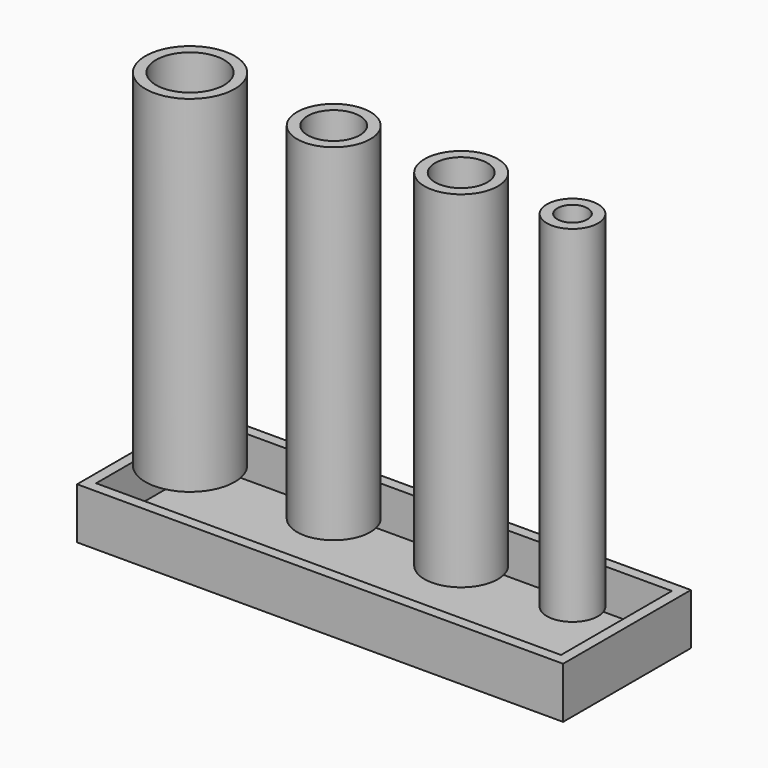
from build123d import *

# Parameters (mm, degrees)
F0_R     = 10.721612753
F1_DEPTH = 83.058
F0_R_2   = 8.8103259694
F0_R_3   = 8.8179558516
F0_R_4   = 6.164722253
F2_W     = 116.6835911572
F2_H     = 12.2901778668
F3_DEPTH = 19.177
F4_T     = -2.54
F4_2_T   = -2.54
F4_3_T   = -2.54
F4_4_T   = -2.54
F5_T     = -2.54


# Not quite as in the source:
# - a feature names something its author has since deleted; it is built from what else it names


with BuildPart() as f1:
    # F0 (on Top) → F1 (new body)
    with BuildSketch(Plane.XY):
        with Locations((-50.1845553517, 0)):
            Circle(F0_R)
    extrude(amount=F1_DEPTH)

    # F4
    f4_openings = [f1.faces().sort_by_distance(p)[0] for p in [
        (-50.184555, 0, 83.058),
    ]]
    offset(amount=F4_T, openings=f4_openings)


with BuildPart() as f1b:
    # F0 (on Top) → F1, piece 2 (new body)
    with BuildSketch(Plane.XY):
        with Locations((-15.6907774508, 0)):
            Circle(F0_R_2)
    extrude(amount=F1_DEPTH)

    # F4#4
    f4_4_openings = [f1b.faces().sort_by_distance(p)[0] for p in [
        (-15.690777, 0, 83.058),
    ]]
    offset(amount=F4_4_T, openings=f4_4_openings)


with BuildPart() as f1c:
    # F0 (on Top) → F1, piece 3 (new body)
    with BuildSketch(Plane.XY):
        with Locations((14.9127244949, 0)):
            Circle(F0_R_3)
    extrude(amount=F1_DEPTH)

    # F4#2
    f4_2_openings = [f1c.faces().sort_by_distance(p)[0] for p in [
        (14.912724, 0, 83.058),
    ]]
    offset(amount=F4_2_T, openings=f4_2_openings)


with BuildPart() as f1d:
    # F0 (on Top) → F1, piece 4 (new body)
    with BuildSketch(Plane.XY):
        with Locations((41.6259467602, 0)):
            Circle(F0_R_4)
    extrude(amount=F1_DEPTH)

    # F4#3
    f4_3_openings = [f1d.faces().sort_by_distance(p)[0] for p in [
        (41.625947, 0, 83.058),
    ]]
    offset(amount=F4_3_T, openings=f4_3_openings)


with BuildPart() as f3:
    # F2 (on Front) → F3 (new body, symmetric)
    with BuildSketch(Plane.XZ):
        with Locations((-3.6206040531, -6.1450889334)):
            Rectangle(F2_W, F2_H)
    extrude(amount=F3_DEPTH, both=True)

    # F5
    f5_openings = [f3.faces().sort_by_distance(p)[0] for p in [
        (-3.620604, 0, 0),
    ]]
    offset(amount=F5_T, openings=f5_openings)


solid = Compound([f1.part, f1b.part, f1c.part, f1d.part, f3.part])
